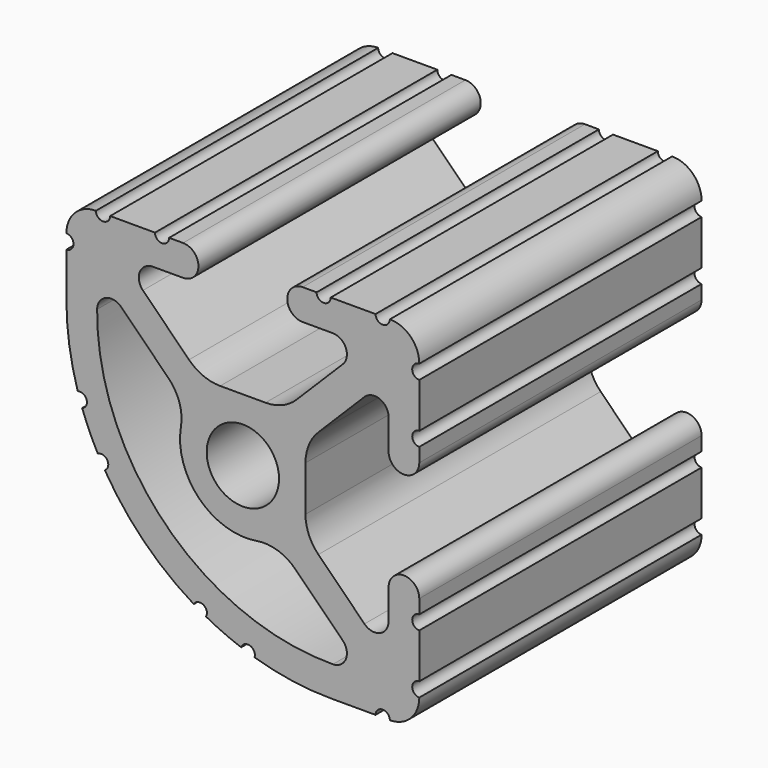
from build123d import *

# Parameters (mm, degrees)
F0_R     = 2.6035
F1_DEPTH = 25.4


# Not quite as in the source:
# - ends of sketch curves that miss each other by under 0.0002 mm in the source are joined


with BuildPart() as f1:
    # F0 (on Front) → F1 (new body)
    with BuildSketch(Plane.XZ):
        with BuildLine():
            ThreePointArc((-12.6999998568, 10.5791116031), (-12.1919492, 10.06475), (-12.6999998568, 9.5503883969))
            Line((-12.6999998568, 9.5503883969), (-12.7, 6.35))
            ThreePointArc((-12.7, 6.35), (-12.4953913266, 3.565448735), (-11.8859605514, 0.8407130437))
            ThreePointArc((-11.8859605514, 0.8407130437), (-11.2503853868, 0.5162584682), (-11.5663491172, -0.1235908641))
            ThreePointArc((-11.5663491172, -0.1235908641), (-11.0492007439, -1.4069525893), (-10.4402782322, -2.6493920286))
            ThreePointArc((-10.4402782322, -2.6493920286), (-9.7531608674, -2.84205605), (-9.9366469283, -3.5316852695))
            ThreePointArc((-9.9366469283, -3.5316852695), (-7.1203841816, -7.1203841816), (-3.5316659689, -9.9366564303))
            ThreePointArc((-3.5316659689, -9.9366564303), (-2.84205605, -9.7531608674), (-2.6494036278, -10.4402857754))
            ThreePointArc((-2.6494036278, -10.4402857754), (-1.4069525893, -11.0492007439), (-0.1235924101, -11.5663361575))
            ThreePointArc((-0.1235924101, -11.5663361575), (0.5162584682, -11.2503853868), (0.8407328825, -11.8859611899))
            ThreePointArc((0.8407328825, -11.8859611899), (3.565448735, -12.4953913266), (6.35, -12.7))
            Line((6.35, -12.7), (9.5504, -12.7))
            ThreePointArc((9.5504, -12.7), (10.06475, -12.1919492), (10.5791116031, -12.6999998568))
            ThreePointArc((10.5791116031, -12.6999998568), (12.0825733161, -12.0825733161), (12.7000122396, -10.579099926))
            ThreePointArc((12.7000122396, -10.579099926), (12.1919492, -10.06475), (12.6999998568, -9.5503883969))
            Line((12.6999998568, -9.5503883969), (12.7, -6.3246))
            ThreePointArc((12.7, -6.3246), (12.192, -5.8166), (12.7, -5.3086))
            Line((12.7, -5.3086), (12.7, -4.3023028))
            ThreePointArc((12.7, -4.3023028), (11.5951, -3.1974028), (10.4902, -4.3023028))
            Line((10.4902, -4.3023028), (10.4902, -6.4747902))
            ThreePointArc((10.4902, -6.4747902), (9.8630063673, -7.413451805), (8.7557795103, -7.1932106897))
            Line((8.7557795103, -7.1932106897), (5.4384448, -3.8758622))
            ThreePointArc((5.4384448, -3.8758622), (4.7501824843, -2.8458268978), (4.5085, -1.630807))
            Line((4.5085, -1.630807), (4.5085, 1.630807))
            ThreePointArc((4.5085, 1.630807), (4.7501824843, 2.8458268978), (5.4384359697, 3.8758710303))
            Line((5.4384359697, 3.8758710303), (8.7557864, 7.1932038))
            ThreePointArc((8.7557864, 7.1932038), (9.8630063673, 7.413451805), (10.4902, 6.4747902))
            Line((10.4902, 6.4747902), (10.4902, 4.3023028))
            ThreePointArc((10.4902, 4.3023028), (11.5951, 3.1974028), (12.7, 4.3023028))
            Line((12.7, 4.3023028), (12.7, 5.3086))
            ThreePointArc((12.7, 5.3086), (12.192, 5.8166), (12.7, 6.3246))
            Line((12.7, 6.3246), (12.7, 9.5504))
            ThreePointArc((12.7, 9.5504), (12.1919492, 10.06475), (12.6999998568, 10.5791116031))
            ThreePointArc((12.6999998568, 10.5791116031), (12.0825733161, 12.0825733161), (10.579099926, 12.7000122396))
            ThreePointArc((10.579099926, 12.7000122396), (10.06475, 12.1919492), (9.5503883969, 12.6999998568))
            Line((9.5503883969, 12.6999998568), (6.3246, 12.7))
            ThreePointArc((6.3246, 12.7), (5.8166, 12.192), (5.3086, 12.7))
            Line((5.3086, 12.7), (4.3023028, 12.7))
            ThreePointArc((4.3023028, 12.7), (3.1974028, 11.5951), (4.3023028, 10.4902))
            Line((4.3023028, 10.4902), (6.4747902, 10.4902))
            ThreePointArc((6.4747902, 10.4902), (7.413451805, 9.8630063673), (7.1932106897, 8.7557795103))
            Line((7.1932106897, 8.7557795103), (3.8758622, 5.4384448))
            ThreePointArc((3.8758622, 5.4384448), (2.8458268978, 4.7501824843), (1.630807, 4.5085))
            Line((1.630807, 4.5085), (-1.630807, 4.5085))
            ThreePointArc((-1.630807, 4.5085), (-2.8458268978, 4.7501824843), (-3.8758710303, 5.4384359697))
            Line((-3.8758710303, 5.4384359697), (-7.1932038, 8.7557864))
            ThreePointArc((-7.1932038, 8.7557864), (-7.413451805, 9.8630063673), (-6.4747902, 10.4902))
            Line((-6.4747902, 10.4902), (-4.3023028, 10.4902))
            ThreePointArc((-4.3023028, 10.4902), (-3.1974028, 11.5951), (-4.3023028, 12.7))
            Line((-4.3023028, 12.7), (-5.3086, 12.7))
            ThreePointArc((-5.3086, 12.7), (-5.8166, 12.192), (-6.3246, 12.7))
            Line((-6.3246, 12.7), (-9.5504, 12.7))
            ThreePointArc((-9.5504, 12.7), (-10.06475, 12.1919492), (-10.5791116031, 12.6999998568))
            ThreePointArc((-10.5791116031, 12.6999998568), (-12.0825733161, 12.0825733161), (-12.6999998568, 10.5791116031))
        make_face()
        with BuildLine():
            ThreePointArc((-10.4896860957, 6.4822831536), (-9.8588365186, 7.4144880425), (-8.7552969103, 7.1927280897))
            Line((-8.7552969103, 7.1927280897), (-5.3427122, 3.7801296))
            ThreePointArc((-5.3427122, 3.7801296), (-4.5640049581, 2.5033128493), (-4.4562086701, 1.0116578151))
            ThreePointArc((-4.4562086701, 1.0116578151), (-3.1300157893, -3.1300157893), (1.0116576108, -4.4562074473))
            ThreePointArc((1.0116576108, -4.4562074473), (2.5033128493, -4.5640049581), (3.7801384303, -5.3427033697))
            Line((3.7801384303, -5.3427033697), (7.1927212, -8.7553038))
            ThreePointArc((7.1927212, -8.7553038), (7.4144880425, -9.8588365186), (6.4822831536, -10.4896860957))
            ThreePointArc((6.4822831536, -10.4896860957), (-5.5578196165, -5.5578196165), (-10.4896860957, 6.4822831536))
        make_face(mode=Mode.SUBTRACT)
        Circle(F0_R, mode=Mode.SUBTRACT)
    extrude(amount=F1_DEPTH)


solid = f1.part
